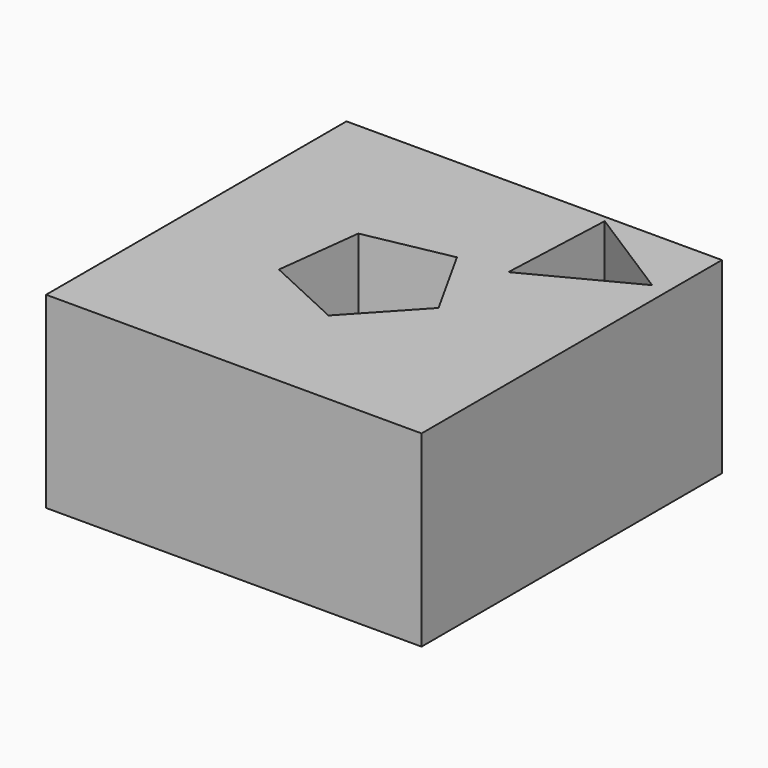
from build123d import *

# Parameters (mm, degrees)
F0_W     = 50.8
F0_H     = 50.8
F1_DEPTH = 25.4
F2_DEPTH = 25.4


# Not quite as in the source:
# - a feature names something its author has since deleted; it is built from what else it names


with BuildPart() as f1:
    # F0 (on Top) → F1 (new body)
    with BuildSketch(Plane.XY):
        with Locations((25.4, -16.6914236449)):
            Rectangle(F0_W, F0_H)
        Polygon((28.5474364771, -8.2873642427), (34.2667401254, -18.5540249534), (26.2699275792, -27.1659785919), (15.6083219757, -22.2217979392), (17.0158998843, -10.5541726109), align=None, mode=Mode.SUBTRACT)
        Polygon((35.5715639889, 7.9258885235), (48.6309623563, -0.3860413606), (34.9029207385, -7.5398471628), align=None, mode=Mode.SUBTRACT)
    extrude(amount=F1_DEPTH)

    # F0 (on Top) → F2 (join)
    with BuildSketch(Plane.XY):
        with Locations((25.4, -16.6914236449)):
            Rectangle(F0_W, F0_H)
        Polygon((28.5474364771, -8.2873642427), (34.2667401254, -18.5540249534), (26.2699275792, -27.1659785919), (15.6083219757, -22.2217979392), (17.0158998843, -10.5541726109), align=None, mode=Mode.SUBTRACT)
        Polygon((35.5715639889, 7.9258885235), (48.6309623563, -0.3860413606), (34.9029207385, -7.5398471628), align=None, mode=Mode.SUBTRACT)
    extrude(amount=F2_DEPTH)


solid = f1.part
